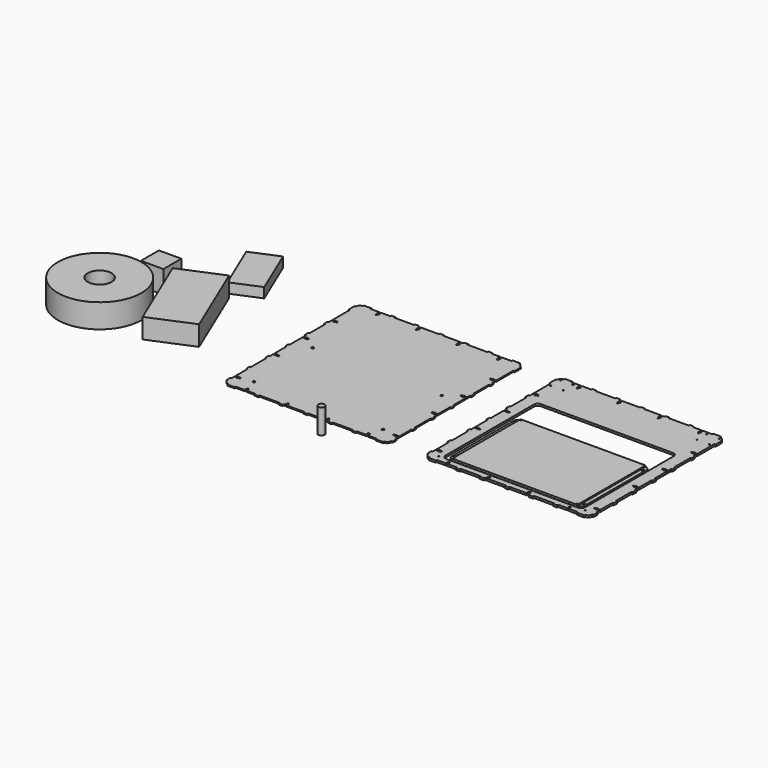
from build123d import *

# Parameters (mm, degrees)
F0_R     = 8
F1_DEPTH = 62
F2_R     = 1.5
F2_R_2   = 50
F2_R_3   = 10
F3_DEPTH = 5
F2_W     = 314
F2_H     = 214
F2_R_4   = 3
F4_DEPTH = 2
F5_DEPTH = 3
F6_DEPTH = 50
F2_R_5   = 105
F2_R_6   = 30
F7_DEPTH = 60
F8_DEPTH = 25
F2_W_2   = 56.4
F2_H_2   = 56.4
F9_DEPTH = 57


with BuildPart() as f1:
    # F0 (on Top) → F1 (new body)
    with BuildSketch(Plane.XY):
        with Locations((-429.197281599, -257.8284740448)):
            Circle(F0_R)
    extrude(amount=F1_DEPTH)


with BuildPart() as f3:
    # F2 (on Top) → F3 (new body)
    with BuildSketch(Plane.XY):
        with BuildLine():
            Line((5, -211.25), (49.3, -211.25))
            Line((49.3, -211.25), (49.3, -208.35))
            Line((49.3, -208.35), (47.8, -208.35))
            Line((47.8, -208.35), (47.8, -205.75))
            Line((47.8, -205.75), (49.3, -205.75))
            Line((49.3, -205.75), (49.3, -202.75))
            Line((49.3, -202.75), (52.7, -202.75))
            Line((52.7, -202.75), (52.7, -205.75))
            Line((52.7, -205.75), (54.2, -205.75))
            Line((54.2, -205.75), (54.2, -208.35))
            Line((54.2, -208.35), (52.7, -208.35))
            Line((52.7, -208.35), (52.7, -211.25))
            Line((52.7, -211.25), (57, -211.25))
            Line((57, -211.25), (57, -214.25))
            Line((57, -214.25), (67, -214.25))
            Line((67, -214.25), (67, -211.25))
            Line((67, -211.25), (117, -211.25))
            Line((117, -211.25), (117, -214.25))
            Line((117, -214.25), (127, -214.25))
            Line((127, -214.25), (127, -211.25))
            Line((127, -211.25), (150.3, -211.25))
            Line((150.3, -211.25), (150.3, -208.35))
            Line((150.3, -208.35), (148.8, -208.35))
            Line((148.8, -208.35), (148.8, -205.75))
            Line((148.8, -205.75), (150.3, -205.75))
            Line((150.3, -205.75), (150.3, -202.75))
            Line((150.3, -202.75), (153.7, -202.75))
            Line((153.7, -202.75), (153.7, -205.75))
            Line((153.7, -205.75), (155.2, -205.75))
            Line((155.2, -205.75), (155.2, -208.35))
            Line((155.2, -208.35), (153.7, -208.35))
            Line((153.7, -208.35), (153.7, -211.25))
            Line((153.7, -211.25), (177, -211.25))
            Line((177, -211.25), (177, -214.25))
            Line((177, -214.25), (195.5, -214.25))
            Line((195.5, -214.25), (195.5, -211.25))
            ThreePointArc((195.5, -211.25), (202.5710678119, -208.3210678119), (205.5, -201.25))
            Line((205.5, -201.25), (208.5, -201.25))
            Line((208.5, -201.25), (208.5, -188.250032))
            Line((208.5, -188.250032), (205.5, -188.250049))
            Line((205.5, -188.250049), (205.5, -179.449994))
            Line((205.5, -179.449994), (199.1, -179.449994))
            Line((199.1, -179.449994), (199.1, -180.949994))
            Line((199.1, -180.949994), (196.5, -180.949994))
            Line((196.5, -180.949994), (196.5, -179.449994))
            Line((196.5, -179.449994), (191.5, -179.449994))
            Line((191.5, -179.449994), (191.5, -176.049994))
            Line((191.5, -176.049994), (196.5, -176.049994))
            Line((196.5, -176.049994), (196.5, -174.549994))
            Line((196.5, -174.549994), (199.1, -174.549994))
            Line((199.1, -174.549994), (199.1, -176.049994))
            Line((199.1, -176.049994), (205.5, -176.049994))
            Line((205.5, -176.049994), (205.5, -138.250065))
            Line((205.5, -138.250065), (208.5, -138.250065))
            Line((208.5, -138.250065), (208.5, -128.250065))
            Line((208.5, -128.250065), (205.5, -128.250065))
            Line((205.5, -128.250065), (205.5, -78.250065))
            Line((205.5, -78.250065), (208.5, -78.250065))
            Line((208.5, -78.250065), (208.5, -68.250065))
            Line((208.5, -68.250065), (205.5, -68.250065))
            Line((205.5, -68.250065), (205.5, -58.449994))
            Line((205.5, -58.449994), (199.1, -58.449994))
            Line((199.1, -58.449994), (199.1, -59.949994))
            Line((199.1, -59.949994), (196.5, -59.949994))
            Line((196.5, -59.949994), (196.5, -58.449994))
            Line((196.5, -58.449994), (191.5, -58.449994))
            Line((191.5, -58.449994), (191.5, -55.049994))
            Line((191.5, -55.049994), (196.5, -55.049994))
            Line((196.5, -55.049994), (196.5, -53.549994))
            Line((196.5, -53.549994), (199.1, -53.549994))
            Line((199.1, -53.549994), (199.1, -55.049994))
            Line((199.1, -55.049994), (205.5, -55.049994))
            Line((205.5, -55.049994), (205.5, -16.250065))
            Line((205.5, -16.250065), (208.5, -16.250065))
            Line((208.5, -16.250065), (208.5, -6.250065))
            Line((208.5, -6.250065), (205.5, -6.250065))
            Line((205.5, -6.250065), (205.5, 33.550006))
            Line((205.5, 33.550006), (199.1, 33.550006))
            Line((199.1, 33.550006), (199.1, 32.050006))
            Line((199.1, 32.050006), (196.5, 32.050006))
            Line((196.5, 32.050006), (196.5, 33.550006))
            Line((196.5, 33.550006), (191.5, 33.550006))
            Line((191.5, 33.550006), (191.5, 36.950006))
            Line((191.5, 36.950006), (196.5, 36.950006))
            Line((196.5, 36.950006), (196.5, 38.450006))
            Line((196.5, 38.450006), (199.1, 38.450006))
            Line((199.1, 38.450006), (199.1, 36.950006))
            Line((199.1, 36.950006), (205.5, 36.950006))
            Line((205.5, 36.950006), (205.5, 45.749935))
            Line((205.5, 45.749935), (208.5, 45.749935))
            Line((208.5, 45.749935), (208.5, 55.749935))
            Line((208.5, 55.749935), (205.5, 55.749935))
            Line((205.5, 55.749935), (205.5, 105.749935))
            Line((205.5, 105.749935), (208.5, 105.749935))
            Line((208.5, 105.749935), (208.5, 115.749935))
            Line((208.5, 115.749935), (205.5, 115.749935))
            Line((205.5, 115.749935), (205.5, 124.550006))
            Line((205.5, 124.550006), (199.1, 124.550006))
            Line((199.1, 124.550006), (199.1, 123.050006))
            Line((199.1, 123.050006), (196.5, 123.050006))
            Line((196.5, 123.050006), (196.5, 124.550006))
            Line((196.5, 124.550006), (191.5, 124.550006))
            Line((191.5, 124.550006), (191.5, 127.950006))
            Line((191.5, 127.950006), (196.5, 127.950006))
            Line((196.5, 127.950006), (196.5, 129.450006))
            Line((196.5, 129.450006), (199.1, 129.450006))
            Line((199.1, 129.450006), (199.1, 127.950006))
            Line((199.1, 127.950006), (205.5, 127.950006))
            Line((205.5, 127.950006), (205.5, 181.25))
            Line((205.5, 181.25), (208.5, 181.25))
            Line((208.5, 181.25), (208.5, 201.25))
            Line((208.5, 201.25), (205.5, 201.25))
            ThreePointArc((205.5, 201.25), (202.5710678119, 208.3210678119), (195.5, 211.25))
            Line((195.5, 211.25), (195.5, 214.25))
            Line((195.5, 214.25), (177, 214.25))
            Line((177, 214.25), (177, 211.25))
            Line((177, 211.25), (153.700002, 211.25))
            Line((153.700002, 211.25), (153.700002, 204.85))
            Line((153.700002, 204.85), (155.200002, 204.85))
            Line((155.200002, 204.85), (155.200002, 202.25))
            Line((155.200002, 202.25), (153.700002, 202.25))
            Line((153.700002, 202.25), (153.700002, 197.25))
            Line((153.700002, 197.25), (150.300002, 197.25))
            Line((150.300002, 197.25), (150.300002, 202.25))
            Line((150.300002, 202.25), (148.800002, 202.25))
            Line((148.800002, 202.25), (148.800002, 204.85))
            Line((148.800002, 204.85), (150.300002, 204.85))
            Line((150.300002, 204.85), (150.300002, 211.25))
            Line((150.300002, 211.25), (127, 211.25))
            Line((127, 211.25), (127, 214.25))
            Line((127, 214.25), (117, 214.25))
            Line((117, 214.25), (117, 211.25))
            Line((117, 211.25), (67, 211.25))
            Line((67, 211.25), (67, 214.25))
            Line((67, 214.25), (57, 214.25))
            Line((57, 214.25), (57, 211.25))
            Line((57, 211.25), (52.700002, 211.25))
            Line((52.700002, 211.25), (52.700002, 204.85))
            Line((52.700002, 204.85), (54.200002, 204.85))
            Line((54.200002, 204.85), (54.200002, 202.25))
            Line((54.200002, 202.25), (52.700002, 202.25))
            Line((52.700002, 202.25), (52.700002, 197.25))
            Line((52.700002, 197.25), (49.300002, 197.25))
            Line((49.300002, 197.25), (49.300002, 202.25))
            Line((49.300002, 202.25), (47.800002, 202.25))
            Line((47.800002, 202.25), (47.800002, 204.85))
            Line((47.800002, 204.85), (49.300002, 204.85))
            Line((49.300002, 204.85), (49.300002, 211.25))
            Line((49.300002, 211.25), (5, 211.25))
            Line((5, 211.25), (5, 214.25))
            Line((5, 214.25), (-5, 214.25))
            Line((-5, 214.25), (-5, 211.25))
            Line((-5, 211.25), (-49.299998, 211.25))
            Line((-49.299998, 211.25), (-49.299998, 204.85))
            Line((-49.299998, 204.85), (-47.799998, 204.85))
            Line((-47.799998, 204.85), (-47.799998, 202.25))
            Line((-47.799998, 202.25), (-49.299998, 202.25))
            Line((-49.299998, 202.25), (-49.299998, 197.25))
            Line((-49.299998, 197.25), (-52.699998, 197.25))
            Line((-52.699998, 197.25), (-52.699998, 202.25))
            Line((-52.699998, 202.25), (-54.199998, 202.25))
            Line((-54.199998, 202.25), (-54.199998, 204.85))
            Line((-54.199998, 204.85), (-52.699998, 204.85))
            Line((-52.699998, 204.85), (-52.699998, 211.25))
            Line((-52.699998, 211.25), (-57, 211.25))
            Line((-57, 211.25), (-57, 214.25))
            Line((-57, 214.25), (-67, 214.25))
            Line((-67, 214.25), (-67, 211.25))
            Line((-67, 211.25), (-117, 211.25))
            Line((-117, 211.25), (-117, 214.25))
            Line((-117, 214.25), (-127, 214.25))
            Line((-127, 214.25), (-127, 211.25))
            Line((-127, 211.25), (-150.299998, 211.25))
            Line((-150.299998, 211.25), (-150.299998, 204.85))
            Line((-150.299998, 204.85), (-148.799998, 204.85))
            Line((-148.799998, 204.85), (-148.799998, 202.25))
            Line((-148.799998, 202.25), (-150.299998, 202.25))
            Line((-150.299998, 202.25), (-150.299998, 197.25))
            Line((-150.299998, 197.25), (-153.699998, 197.25))
            Line((-153.699998, 197.25), (-153.699998, 202.25))
            Line((-153.699998, 202.25), (-155.199998, 202.25))
            Line((-155.199998, 202.25), (-155.199998, 204.85))
            Line((-155.199998, 204.85), (-153.699998, 204.85))
            Line((-153.699998, 204.85), (-153.699998, 211.25))
            Line((-153.699998, 211.25), (-177, 211.25))
            Line((-177, 211.25), (-177, 214.25))
            Line((-177, 214.25), (-195.5, 214.25))
            Line((-195.5, 214.25), (-195.5, 211.25))
            ThreePointArc((-195.5, 211.25), (-202.5710678119, 208.3210678119), (-205.5, 201.25))
            Line((-205.5, 201.25), (-208.5, 201.25))
            Line((-208.5, 201.25), (-208.5, 181.25))
            Line((-208.5, 181.25), (-205.5, 181.25))
            Line((-205.5, 181.25), (-205.5, 127.950006))
            Line((-205.5, 127.950006), (-199.1, 127.950006))
            Line((-199.1, 127.950006), (-199.1, 129.450006))
            Line((-199.1, 129.450006), (-196.5, 129.450006))
            Line((-196.5, 129.450006), (-196.5, 127.950006))
            Line((-196.5, 127.950006), (-191.5, 127.950006))
            Line((-191.5, 127.950006), (-191.5, 124.550006))
            Line((-191.5, 124.550006), (-196.5, 124.550006))
            Line((-196.5, 124.550006), (-196.5, 123.050006))
            Line((-196.5, 123.050006), (-199.1, 123.050006))
            Line((-199.1, 123.050006), (-199.1, 124.550006))
            Line((-199.1, 124.550006), (-205.5, 124.550006))
            Line((-205.5, 124.550006), (-205.5, 115.749935))
            Line((-205.5, 115.749935), (-208.5, 115.749935))
            Line((-208.5, 115.749935), (-208.5, 105.749935))
            Line((-208.5, 105.749935), (-205.5, 105.749935))
            Line((-205.5, 105.749935), (-205.5, 55.749935))
            Line((-205.5, 55.749935), (-208.5, 55.749935))
            Line((-208.5, 55.749935), (-208.5, 45.749935))
            Line((-208.5, 45.749935), (-205.5, 45.749935))
            Line((-205.5, 45.749935), (-205.5, 36.950006))
            Line((-205.5, 36.950006), (-199.1, 36.950006))
            Line((-199.1, 36.950006), (-199.1, 38.450006))
            Line((-199.1, 38.450006), (-196.5, 38.450006))
            Line((-196.5, 38.450006), (-196.5, 36.950006))
            Line((-196.5, 36.950006), (-191.5, 36.950006))
            Line((-191.5, 36.950006), (-191.5, 33.550006))
            Line((-191.5, 33.550006), (-196.5, 33.550006))
            Line((-196.5, 33.550006), (-196.5, 32.050006))
            Line((-196.5, 32.050006), (-199.1, 32.050006))
            Line((-199.1, 32.050006), (-199.1, 33.550006))
            Line((-199.1, 33.550006), (-205.5, 33.550006))
            Line((-205.5, 33.550006), (-205.5, -6.250065))
            Line((-205.5, -6.250065), (-208.5, -6.250065))
            Line((-208.5, -6.250065), (-208.5, -16.250065))
            Line((-208.5, -16.250065), (-205.5, -16.250065))
            Line((-205.5, -16.250065), (-205.5, -55.049994))
            Line((-205.5, -55.049994), (-199.1, -55.049994))
            Line((-199.1, -55.049994), (-199.1, -53.549994))
            Line((-199.1, -53.549994), (-196.5, -53.549994))
            Line((-196.5, -53.549994), (-196.5, -55.049994))
            Line((-196.5, -55.049994), (-191.5, -55.049994))
            Line((-191.5, -55.049994), (-191.5, -58.449994))
            Line((-191.5, -58.449994), (-196.5, -58.449994))
            Line((-196.5, -58.449994), (-196.5, -59.949994))
            Line((-196.5, -59.949994), (-199.1, -59.949994))
            Line((-199.1, -59.949994), (-199.1, -58.449994))
            Line((-199.1, -58.449994), (-205.5, -58.449994))
            Line((-205.5, -58.449994), (-205.5, -68.250065))
            Line((-205.5, -68.250065), (-208.5, -68.250065))
            Line((-208.5, -68.250065), (-208.5, -78.250065))
            Line((-208.5, -78.250065), (-205.5, -78.250065))
            Line((-205.5, -78.250065), (-205.5, -128.250065))
            Line((-205.5, -128.250065), (-208.5, -128.250065))
            Line((-208.5, -128.250065), (-208.5, -138.250065))
            Line((-208.5, -138.250065), (-205.5, -138.250065))
            Line((-205.5, -138.250065), (-205.5, -176.049994))
            Line((-205.5, -176.049994), (-199.1, -176.049994))
            Line((-199.1, -176.049994), (-199.1, -174.549994))
            Line((-199.1, -174.549994), (-196.5, -174.549994))
            Line((-196.5, -174.549994), (-196.5, -176.049994))
            Line((-196.5, -176.049994), (-191.5, -176.049994))
            Line((-191.5, -176.049994), (-191.5, -179.449994))
            Line((-191.5, -179.449994), (-196.5, -179.449994))
            Line((-196.5, -179.449994), (-196.5, -180.949994))
            Line((-196.5, -180.949994), (-199.1, -180.949994))
            Line((-199.1, -180.949994), (-199.1, -179.449994))
            Line((-199.1, -179.449994), (-205.5, -179.449994))
            Line((-205.5, -179.449994), (-205.5, -188.250049))
            Line((-205.5, -188.250049), (-208.5, -188.250032))
            Line((-208.5, -188.250032), (-208.5, -201.25))
            Line((-208.5, -201.25), (-205.5, -201.25))
            ThreePointArc((-205.5, -201.25), (-202.5710678119, -208.3210678119), (-195.5, -211.25))
            Line((-195.5, -211.25), (-195.5, -214.25))
            Line((-195.5, -214.25), (-177, -214.25))
            Line((-177, -214.25), (-177, -211.25))
            Line((-177, -211.25), (-153.7, -211.25))
            Line((-153.7, -211.25), (-153.7, -208.35))
            Line((-153.7, -208.35), (-155.2, -208.35))
            Line((-155.2, -208.35), (-155.2, -205.75))
            Line((-155.2, -205.75), (-153.7, -205.75))
            Line((-153.7, -205.75), (-153.7, -202.75))
            Line((-153.7, -202.75), (-150.3, -202.75))
            Line((-150.3, -202.75), (-150.3, -205.75))
            Line((-150.3, -205.75), (-148.8, -205.75))
            Line((-148.8, -205.75), (-148.8, -208.35))
            Line((-148.8, -208.35), (-150.3, -208.35))
            Line((-150.3, -208.35), (-150.3, -211.25))
            Line((-150.3, -211.25), (-127, -211.25))
            Line((-127, -211.25), (-127, -214.25))
            Line((-127, -214.25), (-117, -214.25))
            Line((-117, -214.25), (-117, -211.25))
            Line((-117, -211.25), (-67, -211.25))
            Line((-67, -211.25), (-67, -214.25))
            Line((-67, -214.25), (-57, -214.25))
            Line((-57, -214.25), (-57, -211.25))
            Line((-57, -211.25), (-52.7, -211.25))
            Line((-52.7, -211.25), (-52.7, -208.35))
            Line((-52.7, -208.35), (-54.2, -208.35))
            Line((-54.2, -208.35), (-54.2, -205.75))
            Line((-54.2, -205.75), (-52.7, -205.75))
            Line((-52.7, -205.75), (-52.7, -202.75))
            Line((-52.7, -202.75), (-49.3, -202.75))
            Line((-49.3, -202.75), (-49.3, -205.75))
            Line((-49.3, -205.75), (-47.8, -205.75))
            Line((-47.8, -205.75), (-47.8, -208.35))
            Line((-47.8, -208.35), (-49.3, -208.35))
            Line((-49.3, -208.35), (-49.3, -211.25))
            Line((-49.3, -211.25), (-5, -211.25))
            Line((-5, -211.25), (-5, -214.25))
            Line((-5, -214.25), (5, -214.25))
            Line((5, -214.25), (5, -211.25))
        make_face()
        with Locations((-183.5, -196.25)):
            Circle(F2_R, mode=Mode.SUBTRACT)
        with Locations((183.5, -196.25)):
            Circle(F2_R, mode=Mode.SUBTRACT)
        with BuildLine():
            ThreePointArc((175.5, -186.25), (172.5710678119, -193.3210678119), (165.5, -196.25))
            Line((165.5, -196.25), (-165.5, -196.25))
            ThreePointArc((-165.5, -196.25), (-172.5710678119, -193.3210678119), (-175.5, -186.25))
            Line((-175.5, -186.25), (-175.5, 91.25))
            ThreePointArc((-175.5, 91.25), (-172.5710678119, 98.3210678119), (-165.5, 101.25))
            Line((-165.5, 101.25), (165.5, 101.25))
            ThreePointArc((165.5, 101.25), (172.5710678119, 98.3210678119), (175.5, 91.25))
            Line((175.5, 91.25), (175.5, -186.25))
        make_face(mode=Mode.SUBTRACT)
        with Locations((-199, 173.75)):
            Circle(F2_R, mode=Mode.SUBTRACT)
        with Locations((-168, 173.75)):
            Circle(F2_R, mode=Mode.SUBTRACT)
        with Locations((-199, 204.75)):
            Circle(F2_R, mode=Mode.SUBTRACT)
        with Locations((-168, 204.75)):
            Circle(F2_R, mode=Mode.SUBTRACT)
        with Locations((-107.5, 156.25)):
            Circle(F2_R_2, mode=Mode.SUBTRACT)
        with Locations((0, 156.25)):
            Circle(F2_R_2, mode=Mode.SUBTRACT)
        with Locations((107.5, 156.25)):
            Circle(F2_R_2, mode=Mode.SUBTRACT)
        with Locations((168, 173.75)):
            Circle(F2_R, mode=Mode.SUBTRACT)
        with Locations((199, 173.75)):
            Circle(F2_R, mode=Mode.SUBTRACT)
        with Locations((168, 204.75)):
            Circle(F2_R, mode=Mode.SUBTRACT)
        with Locations((199, 204.75)):
            Circle(F2_R, mode=Mode.SUBTRACT)
        with Locations((-107.5, 156.25)):
            Circle(F2_R_2)
        with Locations((-107.5, 156.25)):
            Circle(F2_R_3, mode=Mode.SUBTRACT)
        with Locations((107.5, 156.25)):
            Circle(F2_R_2)
        with Locations((107.5, 156.25)):
            Circle(F2_R_3, mode=Mode.SUBTRACT)
        with Locations((0, 156.25)):
            Circle(F2_R_2)
        with Locations((0, 156.25)):
            Circle(F2_R_3, mode=Mode.SUBTRACT)
        with Locations((-107.5, 156.25)):
            Circle(F2_R_3)
        with Locations((0, 156.25)):
            Circle(F2_R_3)
        with Locations((107.5, 156.25)):
            Circle(F2_R_3)
    extrude(amount=F3_DEPTH)


with BuildPart() as f3b:
    # F2 (on Top) → F3, piece 2 (new body)
    with BuildSketch(Plane.XY):
        with Locations((0, -80.75)):
            Rectangle(F2_W, F2_H)
        with Locations((-154.5, -185.25)):
            Circle(F2_R, mode=Mode.SUBTRACT)
        with Locations((154.5, -185.25)):
            Circle(F2_R, mode=Mode.SUBTRACT)
        with Locations((-154.5, 23.75)):
            Circle(F2_R, mode=Mode.SUBTRACT)
        with Locations((154.5, 23.75)):
            Circle(F2_R, mode=Mode.SUBTRACT)
    extrude(amount=F3_DEPTH)

    # F2 (on Top) → F4 (join)
    with BuildSketch(Plane.XY):
        with BuildLine():
            ThreePointArc((-157, 26.25), (-164.0710678119, 23.3210678119), (-167, 16.25))
            Line((-167, 16.25), (-167, -177.75))
            ThreePointArc((-167, -177.75), (-164.0710678119, -184.8210678119), (-157, -187.75))
            Line((-157, -187.75), (-157, 26.25))
        make_face()
        with Locations((-162, -172.75)):
            Circle(F2_R_4, mode=Mode.SUBTRACT)
        with Locations((-162, 11.25)):
            Circle(F2_R_4, mode=Mode.SUBTRACT)
        with BuildLine():
            ThreePointArc((167, 16.25), (164.0710678119, 23.3210678119), (157, 26.25))
            Line((157, 26.25), (157, -187.75))
            ThreePointArc((157, -187.75), (164.0710678119, -184.8210678119), (167, -177.75))
            Line((167, -177.75), (167, 16.25))
        make_face()
        with Locations((162, -172.75)):
            Circle(F2_R_4, mode=Mode.SUBTRACT)
        with Locations((162, 11.25)):
            Circle(F2_R_4, mode=Mode.SUBTRACT)
    extrude(amount=F4_DEPTH)


with BuildPart() as f5:
    # F2 (on Top) → F5 (new body)
    with BuildSketch(Plane.XY):
        with BuildLine():
            Line((-499.6031921292, -211.2499983311), (-455.3031921292, -211.2499983311))
            Line((-455.3031921292, -211.2499983311), (-455.3031921292, -208.3499983311))
            Line((-455.3031921292, -208.3499983311), (-456.8031921292, -208.3499983311))
            Line((-456.8031921292, -208.3499983311), (-456.8031921292, -205.7499983311))
            Line((-456.8031921292, -205.7499983311), (-455.3031921292, -205.7499983311))
            Line((-455.3031921292, -205.7499983311), (-455.3031921292, -202.7499983311))
            Line((-455.3031921292, -202.7499983311), (-451.9031921292, -202.7499983311))
            Line((-451.9031921292, -202.7499983311), (-451.9031921292, -205.7499983311))
            Line((-451.9031921292, -205.7499983311), (-450.4031921292, -205.7499983311))
            Line((-450.4031921292, -205.7499983311), (-450.4031921292, -208.3499983311))
            Line((-450.4031921292, -208.3499983311), (-451.9031921292, -208.3499983311))
            Line((-451.9031921292, -208.3499983311), (-451.9031921292, -211.2499983311))
            Line((-451.9031921292, -211.2499983311), (-447.6031921292, -211.2499983311))
            Line((-447.6031921292, -211.2499983311), (-447.6031921292, -214.2499983311))
            Line((-447.6031921292, -214.2499983311), (-437.6031921292, -214.2499983311))
            Line((-437.6031921292, -214.2499983311), (-437.6031921292, -211.2499983311))
            Line((-437.6031921292, -211.2499983311), (-387.6031921292, -211.2499983311))
            Line((-387.6031921292, -211.2499983311), (-387.6031921292, -214.2499983311))
            Line((-387.6031921292, -214.2499983311), (-377.6031921292, -214.2499983311))
            Line((-377.6031921292, -214.2499983311), (-377.6031921292, -211.2499983311))
            Line((-377.6031921292, -211.2499983311), (-354.3031921292, -211.2499983311))
            Line((-354.3031921292, -211.2499983311), (-354.3031921292, -208.3499983311))
            Line((-354.3031921292, -208.3499983311), (-355.8031921292, -208.3499983311))
            Line((-355.8031921292, -208.3499983311), (-355.8031921292, -205.7499983311))
            Line((-355.8031921292, -205.7499983311), (-354.3031921292, -205.7499983311))
            Line((-354.3031921292, -205.7499983311), (-354.3031921292, -202.7499983311))
            Line((-354.3031921292, -202.7499983311), (-350.9031921292, -202.7499983311))
            Line((-350.9031921292, -202.7499983311), (-350.9031921292, -205.7499983311))
            Line((-350.9031921292, -205.7499983311), (-349.4031921292, -205.7499983311))
            Line((-349.4031921292, -205.7499983311), (-349.4031921292, -208.3499983311))
            Line((-349.4031921292, -208.3499983311), (-350.9031921292, -208.3499983311))
            Line((-350.9031921292, -208.3499983311), (-350.9031921292, -211.2499983311))
            Line((-350.9031921292, -211.2499983311), (-327.6031921292, -211.2499983311))
            Line((-327.6031921292, -211.2499983311), (-327.6031921292, -214.2499983311))
            Line((-327.6031921292, -214.2499983311), (-309.1031921292, -214.2499983311))
            Line((-309.1031921292, -214.2499983311), (-309.1031921292, -211.2499983311))
            ThreePointArc((-309.1031921292, -211.2499983311), (-302.0321243174, -208.3210661429), (-299.1031921292, -201.2499983311))
            Line((-299.1031921292, -201.2499983311), (-296.1031921292, -201.2499983311))
            Line((-296.1031921292, -201.2499983311), (-296.1031921292, -188.2500303311))
            Line((-296.1031921292, -188.2500303311), (-299.1031921292, -188.2500473311))
            Line((-299.1031921292, -188.2500473311), (-299.1031921292, -179.4499923311))
            Line((-299.1031921292, -179.4499923311), (-305.5031921292, -179.4499923311))
            Line((-305.5031921292, -179.4499923311), (-305.5031921292, -180.9499923311))
            Line((-305.5031921292, -180.9499923311), (-308.1031921292, -180.9499923311))
            Line((-308.1031921292, -180.9499923311), (-308.1031921292, -179.4499923311))
            Line((-308.1031921292, -179.4499923311), (-313.1031921292, -179.4499923311))
            Line((-313.1031921292, -179.4499923311), (-313.1031921292, -176.0499923311))
            Line((-313.1031921292, -176.0499923311), (-308.1031921292, -176.0499923311))
            Line((-308.1031921292, -176.0499923311), (-308.1031921292, -174.5499923311))
            Line((-308.1031921292, -174.5499923311), (-305.5031921292, -174.5499923311))
            Line((-305.5031921292, -174.5499923311), (-305.5031921292, -176.0499923311))
            Line((-305.5031921292, -176.0499923311), (-299.1031921292, -176.0499923311))
            Line((-299.1031921292, -176.0499923311), (-299.1031921292, -138.2500633311))
            Line((-299.1031921292, -138.2500633311), (-296.1031921292, -138.2500633311))
            Line((-296.1031921292, -138.2500633311), (-296.1031921292, -128.2500633311))
            Line((-296.1031921292, -128.2500633311), (-299.1031921292, -128.2500633311))
            Line((-299.1031921292, -128.2500633311), (-299.1031921292, -78.2500633311))
            Line((-299.1031921292, -78.2500633311), (-296.1031921292, -78.2500633311))
            Line((-296.1031921292, -78.2500633311), (-296.1031921292, -68.2500633311))
            Line((-296.1031921292, -68.2500633311), (-299.1031921292, -68.2500633311))
            Line((-299.1031921292, -68.2500633311), (-299.1031921292, -58.4499923311))
            Line((-299.1031921292, -58.4499923311), (-305.5031921292, -58.4499923311))
            Line((-305.5031921292, -58.4499923311), (-305.5031921292, -59.9499923311))
            Line((-305.5031921292, -59.9499923311), (-308.1031921292, -59.9499923311))
            Line((-308.1031921292, -59.9499923311), (-308.1031921292, -58.4499923311))
            Line((-308.1031921292, -58.4499923311), (-313.1031921292, -58.4499923311))
            Line((-313.1031921292, -58.4499923311), (-313.1031921292, -55.0499923311))
            Line((-313.1031921292, -55.0499923311), (-308.1031921292, -55.0499923311))
            Line((-308.1031921292, -55.0499923311), (-308.1031921292, -53.5499923311))
            Line((-308.1031921292, -53.5499923311), (-305.5031921292, -53.5499923311))
            Line((-305.5031921292, -53.5499923311), (-305.5031921292, -55.0499923311))
            Line((-305.5031921292, -55.0499923311), (-299.1031921292, -55.0499923311))
            Line((-299.1031921292, -55.0499923311), (-299.1031921292, -16.2500633311))
            Line((-299.1031921292, -16.2500633311), (-296.1031921292, -16.2500633311))
            Line((-296.1031921292, -16.2500633311), (-296.1031921292, -6.2500633311))
            Line((-296.1031921292, -6.2500633311), (-299.1031921292, -6.2500633311))
            Line((-299.1031921292, -6.2500633311), (-299.1031921292, 33.5500076689))
            Line((-299.1031921292, 33.5500076689), (-305.5031921292, 33.5500076689))
            Line((-305.5031921292, 33.5500076689), (-305.5031921292, 32.0500076689))
            Line((-305.5031921292, 32.0500076689), (-308.1031921292, 32.0500076689))
            Line((-308.1031921292, 32.0500076689), (-308.1031921292, 33.5500076689))
            Line((-308.1031921292, 33.5500076689), (-313.1031921292, 33.5500076689))
            Line((-313.1031921292, 33.5500076689), (-313.1031921292, 36.9500076689))
            Line((-313.1031921292, 36.9500076689), (-308.1031921292, 36.9500076689))
            Line((-308.1031921292, 36.9500076689), (-308.1031921292, 38.4500076689))
            Line((-308.1031921292, 38.4500076689), (-305.5031921292, 38.4500076689))
            Line((-305.5031921292, 38.4500076689), (-305.5031921292, 36.9500076689))
            Line((-305.5031921292, 36.9500076689), (-299.1031921292, 36.9500076689))
            Line((-299.1031921292, 36.9500076689), (-299.1031921292, 45.7499366689))
            Line((-299.1031921292, 45.7499366689), (-296.1031921292, 45.7499366689))
            Line((-296.1031921292, 45.7499366689), (-296.1031921292, 55.7499366689))
            Line((-296.1031921292, 55.7499366689), (-299.1031921292, 55.7499366689))
            Line((-299.1031921292, 55.7499366689), (-299.1031921292, 105.7499366689))
            Line((-299.1031921292, 105.7499366689), (-296.1031921292, 105.7499366689))
            Line((-296.1031921292, 105.7499366689), (-296.1031921292, 115.7499366689))
            Line((-296.1031921292, 115.7499366689), (-299.1031921292, 115.7499366689))
            Line((-299.1031921292, 115.7499366689), (-299.1031921292, 124.5500076689))
            Line((-299.1031921292, 124.5500076689), (-305.5031921292, 124.5500076689))
            Line((-305.5031921292, 124.5500076689), (-305.5031921292, 123.0500076689))
            Line((-305.5031921292, 123.0500076689), (-308.1031921292, 123.0500076689))
            Line((-308.1031921292, 123.0500076689), (-308.1031921292, 124.5500076689))
            Line((-308.1031921292, 124.5500076689), (-313.1031921292, 124.5500076689))
            Line((-313.1031921292, 124.5500076689), (-313.1031921292, 127.9500076689))
            Line((-313.1031921292, 127.9500076689), (-308.1031921292, 127.9500076689))
            Line((-308.1031921292, 127.9500076689), (-308.1031921292, 129.4500076689))
            Line((-308.1031921292, 129.4500076689), (-305.5031921292, 129.4500076689))
            Line((-305.5031921292, 129.4500076689), (-305.5031921292, 127.9500076689))
            Line((-305.5031921292, 127.9500076689), (-299.1031921292, 127.9500076689))
            Line((-299.1031921292, 127.9500076689), (-299.1031921292, 181.2500016689))
            Line((-299.1031921292, 181.2500016689), (-296.1031921292, 181.2500016689))
            Line((-296.1031921292, 181.2500016689), (-296.1031921292, 201.2500016689))
            Line((-296.1031921292, 201.2500016689), (-299.1031921292, 201.2500016689))
            ThreePointArc((-299.1031921292, 201.2500016689), (-302.0321243174, 208.3210694808), (-309.1031921292, 211.2500016689))
            Line((-309.1031921292, 211.2500016689), (-309.1031921292, 214.2500016689))
            Line((-309.1031921292, 214.2500016689), (-327.6031921292, 214.2500016689))
            Line((-327.6031921292, 214.2500016689), (-327.6031921292, 211.2500016689))
            Line((-327.6031921292, 211.2500016689), (-350.9031901292, 211.2500016689))
            Line((-350.9031901292, 211.2500016689), (-350.9031901292, 204.8500016689))
            Line((-350.9031901292, 204.8500016689), (-349.4031901292, 204.8500016689))
            Line((-349.4031901292, 204.8500016689), (-349.4031901292, 202.2500016689))
            Line((-349.4031901292, 202.2500016689), (-350.9031901292, 202.2500016689))
            Line((-350.9031901292, 202.2500016689), (-350.9031901292, 197.2500016689))
            Line((-350.9031901292, 197.2500016689), (-354.3031901292, 197.2500016689))
            Line((-354.3031901292, 197.2500016689), (-354.3031901292, 202.2500016689))
            Line((-354.3031901292, 202.2500016689), (-355.8031901292, 202.2500016689))
            Line((-355.8031901292, 202.2500016689), (-355.8031901292, 204.8500016689))
            Line((-355.8031901292, 204.8500016689), (-354.3031901292, 204.8500016689))
            Line((-354.3031901292, 204.8500016689), (-354.3031901292, 211.2500016689))
            Line((-354.3031901292, 211.2500016689), (-377.6031921292, 211.2500016689))
            Line((-377.6031921292, 211.2500016689), (-377.6031921292, 214.2500016689))
            Line((-377.6031921292, 214.2500016689), (-387.6031921292, 214.2500016689))
            Line((-387.6031921292, 214.2500016689), (-387.6031921292, 211.2500016689))
            Line((-387.6031921292, 211.2500016689), (-437.6031921292, 211.2500016689))
            Line((-437.6031921292, 211.2500016689), (-437.6031921292, 214.2500016689))
            Line((-437.6031921292, 214.2500016689), (-447.6031921292, 214.2500016689))
            Line((-447.6031921292, 214.2500016689), (-447.6031921292, 211.2500016689))
            Line((-447.6031921292, 211.2500016689), (-451.9031901292, 211.2500016689))
            Line((-451.9031901292, 211.2500016689), (-451.9031901292, 204.8500016689))
            Line((-451.9031901292, 204.8500016689), (-450.4031901292, 204.8500016689))
            Line((-450.4031901292, 204.8500016689), (-450.4031901292, 202.2500016689))
            Line((-450.4031901292, 202.2500016689), (-451.9031901292, 202.2500016689))
            Line((-451.9031901292, 202.2500016689), (-451.9031901292, 197.2500016689))
            Line((-451.9031901292, 197.2500016689), (-455.3031901292, 197.2500016689))
            Line((-455.3031901292, 197.2500016689), (-455.3031901292, 202.2500016689))
            Line((-455.3031901292, 202.2500016689), (-456.8031901292, 202.2500016689))
            Line((-456.8031901292, 202.2500016689), (-456.8031901292, 204.8500016689))
            Line((-456.8031901292, 204.8500016689), (-455.3031901292, 204.8500016689))
            Line((-455.3031901292, 204.8500016689), (-455.3031901292, 211.2500016689))
            Line((-455.3031901292, 211.2500016689), (-499.6031921292, 211.2500016689))
            Line((-499.6031921292, 211.2500016689), (-499.6031921292, 214.2500016689))
            Line((-499.6031921292, 214.2500016689), (-509.6031921292, 214.2500016689))
            Line((-509.6031921292, 214.2500016689), (-509.6031921292, 211.2500016689))
            Line((-509.6031921292, 211.2500016689), (-553.9031901292, 211.2500016689))
            Line((-553.9031901292, 211.2500016689), (-553.9031901292, 204.8500016689))
            Line((-553.9031901292, 204.8500016689), (-552.4031901292, 204.8500016689))
            Line((-552.4031901292, 204.8500016689), (-552.4031901292, 202.2500016689))
            Line((-552.4031901292, 202.2500016689), (-553.9031901292, 202.2500016689))
            Line((-553.9031901292, 202.2500016689), (-553.9031901292, 197.2500016689))
            Line((-553.9031901292, 197.2500016689), (-557.3031901292, 197.2500016689))
            Line((-557.3031901292, 197.2500016689), (-557.3031901292, 202.2500016689))
            Line((-557.3031901292, 202.2500016689), (-558.8031901292, 202.2500016689))
            Line((-558.8031901292, 202.2500016689), (-558.8031901292, 204.8500016689))
            Line((-558.8031901292, 204.8500016689), (-557.3031901292, 204.8500016689))
            Line((-557.3031901292, 204.8500016689), (-557.3031901292, 211.2500016689))
            Line((-557.3031901292, 211.2500016689), (-561.6031921292, 211.2500016689))
            Line((-561.6031921292, 211.2500016689), (-561.6031921292, 214.2500016689))
            Line((-561.6031921292, 214.2500016689), (-571.6031921292, 214.2500016689))
            Line((-571.6031921292, 214.2500016689), (-571.6031921292, 211.2500016689))
            Line((-571.6031921292, 211.2500016689), (-621.6031921292, 211.2500016689))
            Line((-621.6031921292, 211.2500016689), (-621.6031921292, 214.2500016689))
            Line((-621.6031921292, 214.2500016689), (-631.6031921292, 214.2500016689))
            Line((-631.6031921292, 214.2500016689), (-631.6031921292, 211.2500016689))
            Line((-631.6031921292, 211.2500016689), (-654.9031901292, 211.2500016689))
            Line((-654.9031901292, 211.2500016689), (-654.9031901292, 204.8500016689))
            Line((-654.9031901292, 204.8500016689), (-653.4031901292, 204.8500016689))
            Line((-653.4031901292, 204.8500016689), (-653.4031901292, 202.2500016689))
            Line((-653.4031901292, 202.2500016689), (-654.9031901292, 202.2500016689))
            Line((-654.9031901292, 202.2500016689), (-654.9031901292, 197.2500016689))
            Line((-654.9031901292, 197.2500016689), (-658.3031901292, 197.2500016689))
            Line((-658.3031901292, 197.2500016689), (-658.3031901292, 202.2500016689))
            Line((-658.3031901292, 202.2500016689), (-659.8031901292, 202.2500016689))
            Line((-659.8031901292, 202.2500016689), (-659.8031901292, 204.8500016689))
            Line((-659.8031901292, 204.8500016689), (-658.3031901292, 204.8500016689))
            Line((-658.3031901292, 204.8500016689), (-658.3031901292, 211.2500016689))
            Line((-658.3031901292, 211.2500016689), (-681.6031921292, 211.2500016689))
            Line((-681.6031921292, 211.2500016689), (-681.6031921292, 214.2500016689))
            Line((-681.6031921292, 214.2500016689), (-700.1031921292, 214.2500016689))
            Line((-700.1031921292, 214.2500016689), (-700.1031921292, 211.2500016689))
            ThreePointArc((-700.1031921292, 211.2500016689), (-707.1742599411, 208.3210694808), (-710.1031921292, 201.2500016689))
            Line((-710.1031921292, 201.2500016689), (-713.1031921292, 201.2500016689))
            Line((-713.1031921292, 201.2500016689), (-713.1031921292, 181.2500016689))
            Line((-713.1031921292, 181.2500016689), (-710.1031921292, 181.2500016689))
            Line((-710.1031921292, 181.2500016689), (-710.1031921292, 127.9500076689))
            Line((-710.1031921292, 127.9500076689), (-703.7031921292, 127.9500076689))
            Line((-703.7031921292, 127.9500076689), (-703.7031921292, 129.4500076689))
            Line((-703.7031921292, 129.4500076689), (-701.1031921292, 129.4500076689))
            Line((-701.1031921292, 129.4500076689), (-701.1031921292, 127.9500076689))
            Line((-701.1031921292, 127.9500076689), (-696.1031921292, 127.9500076689))
            Line((-696.1031921292, 127.9500076689), (-696.1031921292, 124.5500076689))
            Line((-696.1031921292, 124.5500076689), (-701.1031921292, 124.5500076689))
            Line((-701.1031921292, 124.5500076689), (-701.1031921292, 123.0500076689))
            Line((-701.1031921292, 123.0500076689), (-703.7031921292, 123.0500076689))
            Line((-703.7031921292, 123.0500076689), (-703.7031921292, 124.5500076689))
            Line((-703.7031921292, 124.5500076689), (-710.1031921292, 124.5500076689))
            Line((-710.1031921292, 124.5500076689), (-710.1031921292, 115.7499366689))
            Line((-710.1031921292, 115.7499366689), (-713.1031921292, 115.7499366689))
            Line((-713.1031921292, 115.7499366689), (-713.1031921292, 105.7499366689))
            Line((-713.1031921292, 105.7499366689), (-710.1031921292, 105.7499366689))
            Line((-710.1031921292, 105.7499366689), (-710.1031921292, 55.7499366689))
            Line((-710.1031921292, 55.7499366689), (-713.1031921292, 55.7499366689))
            Line((-713.1031921292, 55.7499366689), (-713.1031921292, 45.7499366689))
            Line((-713.1031921292, 45.7499366689), (-710.1031921292, 45.7499366689))
            Line((-710.1031921292, 45.7499366689), (-710.1031921292, 36.9500076689))
            Line((-710.1031921292, 36.9500076689), (-703.7031921292, 36.9500076689))
            Line((-703.7031921292, 36.9500076689), (-703.7031921292, 38.4500076689))
            Line((-703.7031921292, 38.4500076689), (-701.1031921292, 38.4500076689))
            Line((-701.1031921292, 38.4500076689), (-701.1031921292, 36.9500076689))
            Line((-701.1031921292, 36.9500076689), (-696.1031921292, 36.9500076689))
            Line((-696.1031921292, 36.9500076689), (-696.1031921292, 33.5500076689))
            Line((-696.1031921292, 33.5500076689), (-701.1031921292, 33.5500076689))
            Line((-701.1031921292, 33.5500076689), (-701.1031921292, 32.0500076689))
            Line((-701.1031921292, 32.0500076689), (-703.7031921292, 32.0500076689))
            Line((-703.7031921292, 32.0500076689), (-703.7031921292, 33.5500076689))
            Line((-703.7031921292, 33.5500076689), (-710.1031921292, 33.5500076689))
            Line((-710.1031921292, 33.5500076689), (-710.1031921292, -6.2500633311))
            Line((-710.1031921292, -6.2500633311), (-713.1031921292, -6.2500633311))
            Line((-713.1031921292, -6.2500633311), (-713.1031921292, -16.2500633311))
            Line((-713.1031921292, -16.2500633311), (-710.1031921292, -16.2500633311))
            Line((-710.1031921292, -16.2500633311), (-710.1031921292, -55.0499923311))
            Line((-710.1031921292, -55.0499923311), (-703.7031921292, -55.0499923311))
            Line((-703.7031921292, -55.0499923311), (-703.7031921292, -53.5499923311))
            Line((-703.7031921292, -53.5499923311), (-701.1031921292, -53.5499923311))
            Line((-701.1031921292, -53.5499923311), (-701.1031921292, -55.0499923311))
            Line((-701.1031921292, -55.0499923311), (-696.1031921292, -55.0499923311))
            Line((-696.1031921292, -55.0499923311), (-696.1031921292, -58.4499923311))
            Line((-696.1031921292, -58.4499923311), (-701.1031921292, -58.4499923311))
            Line((-701.1031921292, -58.4499923311), (-701.1031921292, -59.9499923311))
            Line((-701.1031921292, -59.9499923311), (-703.7031921292, -59.9499923311))
            Line((-703.7031921292, -59.9499923311), (-703.7031921292, -58.4499923311))
            Line((-703.7031921292, -58.4499923311), (-710.1031921292, -58.4499923311))
            Line((-710.1031921292, -58.4499923311), (-710.1031921292, -68.2500633311))
            Line((-710.1031921292, -68.2500633311), (-713.1031921292, -68.2500633311))
            Line((-713.1031921292, -68.2500633311), (-713.1031921292, -78.2500633311))
            Line((-713.1031921292, -78.2500633311), (-710.1031921292, -78.2500633311))
            Line((-710.1031921292, -78.2500633311), (-710.1031921292, -128.2500633311))
            Line((-710.1031921292, -128.2500633311), (-713.1031921292, -128.2500633311))
            Line((-713.1031921292, -128.2500633311), (-713.1031921292, -138.2500633311))
            Line((-713.1031921292, -138.2500633311), (-710.1031921292, -138.2500633311))
            Line((-710.1031921292, -138.2500633311), (-710.1031921292, -176.0499923311))
            Line((-710.1031921292, -176.0499923311), (-703.7031921292, -176.0499923311))
            Line((-703.7031921292, -176.0499923311), (-703.7031921292, -174.5499923311))
            Line((-703.7031921292, -174.5499923311), (-701.1031921292, -174.5499923311))
            Line((-701.1031921292, -174.5499923311), (-701.1031921292, -176.0499923311))
            Line((-701.1031921292, -176.0499923311), (-696.1031921292, -176.0499923311))
            Line((-696.1031921292, -176.0499923311), (-696.1031921292, -179.4499923311))
            Line((-696.1031921292, -179.4499923311), (-701.1031921292, -179.4499923311))
            Line((-701.1031921292, -179.4499923311), (-701.1031921292, -180.9499923311))
            Line((-701.1031921292, -180.9499923311), (-703.7031921292, -180.9499923311))
            Line((-703.7031921292, -180.9499923311), (-703.7031921292, -179.4499923311))
            Line((-703.7031921292, -179.4499923311), (-710.1031921292, -179.4499923311))
            Line((-710.1031921292, -179.4499923311), (-710.1031921292, -188.2500473311))
            Line((-710.1031921292, -188.2500473311), (-713.1031921292, -188.2500303311))
            Line((-713.1031921292, -188.2500303311), (-713.1031921292, -201.2499983311))
            Line((-713.1031921292, -201.2499983311), (-710.1031921292, -201.2499983311))
            ThreePointArc((-710.1031921292, -201.2499983311), (-707.1742599411, -208.3210661429), (-700.1031921292, -211.2499983311))
            Line((-700.1031921292, -211.2499983311), (-700.1031921292, -214.2499983311))
            Line((-700.1031921292, -214.2499983311), (-681.6031921292, -214.2499983311))
            Line((-681.6031921292, -214.2499983311), (-681.6031921292, -211.2499983311))
            Line((-681.6031921292, -211.2499983311), (-658.3031921292, -211.2499983311))
            Line((-658.3031921292, -211.2499983311), (-658.3031921292, -208.3499983311))
            Line((-658.3031921292, -208.3499983311), (-659.8031921292, -208.3499983311))
            Line((-659.8031921292, -208.3499983311), (-659.8031921292, -205.7499983311))
            Line((-659.8031921292, -205.7499983311), (-658.3031921292, -205.7499983311))
            Line((-658.3031921292, -205.7499983311), (-658.3031921292, -202.7499983311))
            Line((-658.3031921292, -202.7499983311), (-654.9031921292, -202.7499983311))
            Line((-654.9031921292, -202.7499983311), (-654.9031921292, -205.7499983311))
            Line((-654.9031921292, -205.7499983311), (-653.4031921292, -205.7499983311))
            Line((-653.4031921292, -205.7499983311), (-653.4031921292, -208.3499983311))
            Line((-653.4031921292, -208.3499983311), (-654.9031921292, -208.3499983311))
            Line((-654.9031921292, -208.3499983311), (-654.9031921292, -211.2499983311))
            Line((-654.9031921292, -211.2499983311), (-631.6031921292, -211.2499983311))
            Line((-631.6031921292, -211.2499983311), (-631.6031921292, -214.2499983311))
            Line((-631.6031921292, -214.2499983311), (-621.6031921292, -214.2499983311))
            Line((-621.6031921292, -214.2499983311), (-621.6031921292, -211.2499983311))
            Line((-621.6031921292, -211.2499983311), (-571.6031921292, -211.2499983311))
            Line((-571.6031921292, -211.2499983311), (-571.6031921292, -214.2499983311))
            Line((-571.6031921292, -214.2499983311), (-561.6031921292, -214.2499983311))
            Line((-561.6031921292, -214.2499983311), (-561.6031921292, -211.2499983311))
            Line((-561.6031921292, -211.2499983311), (-557.3031921292, -211.2499983311))
            Line((-557.3031921292, -211.2499983311), (-557.3031921292, -208.3499983311))
            Line((-557.3031921292, -208.3499983311), (-558.8031921292, -208.3499983311))
            Line((-558.8031921292, -208.3499983311), (-558.8031921292, -205.7499983311))
            Line((-558.8031921292, -205.7499983311), (-557.3031921292, -205.7499983311))
            Line((-557.3031921292, -205.7499983311), (-557.3031921292, -202.7499983311))
            Line((-557.3031921292, -202.7499983311), (-553.9031921292, -202.7499983311))
            Line((-553.9031921292, -202.7499983311), (-553.9031921292, -205.7499983311))
            Line((-553.9031921292, -205.7499983311), (-552.4031921292, -205.7499983311))
            Line((-552.4031921292, -205.7499983311), (-552.4031921292, -208.3499983311))
            Line((-552.4031921292, -208.3499983311), (-553.9031921292, -208.3499983311))
            Line((-553.9031921292, -208.3499983311), (-553.9031921292, -211.2499983311))
            Line((-553.9031921292, -211.2499983311), (-509.6031921292, -211.2499983311))
            Line((-509.6031921292, -211.2499983311), (-509.6031921292, -214.2499983311))
            Line((-509.6031921292, -214.2499983311), (-499.6031921292, -214.2499983311))
            Line((-499.6031921292, -214.2499983311), (-499.6031921292, -211.2499983311))
        make_face()
        with Locations((-666.6031921292, -172.7499983311)):
            Circle(F2_R_4, mode=Mode.SUBTRACT)
        with Locations((-666.6031921292, 11.2500016689)):
            Circle(F2_R_4, mode=Mode.SUBTRACT)
        with Locations((-342.6031921292, -172.7499983311)):
            Circle(F2_R_4, mode=Mode.SUBTRACT)
        with Locations((-342.6031921292, 11.2500016689)):
            Circle(F2_R_4, mode=Mode.SUBTRACT)
        with Locations((-612.1031921292, 156.2500016689)):
            Circle(F2_R_2, mode=Mode.SUBTRACT)
        with Locations((-504.6031921292, 156.2500016689)):
            Circle(F2_R_2, mode=Mode.SUBTRACT)
        with Locations((-397.1031921292, 156.2500016689)):
            Circle(F2_R_2, mode=Mode.SUBTRACT)
        with Locations((-612.1031921292, 156.2500016689)):
            Circle(F2_R_2)
        with Locations((-612.1031921292, 156.2500016689)):
            Circle(F2_R_3, mode=Mode.SUBTRACT)
        with Locations((-504.6031921292, 156.2500016689)):
            Circle(F2_R_2)
        with Locations((-504.6031921292, 156.2500016689)):
            Circle(F2_R_3, mode=Mode.SUBTRACT)
        with Locations((-397.1031921292, 156.2500016689)):
            Circle(F2_R_2)
        with Locations((-397.1031921292, 156.2500016689)):
            Circle(F2_R_3, mode=Mode.SUBTRACT)
        with Locations((-397.1031921292, 156.2500016689)):
            Circle(F2_R_3)
        with Locations((-504.6031921292, 156.2500016689)):
            Circle(F2_R_3)
        with Locations((-612.1031921292, 156.2500016689)):
            Circle(F2_R_3)
    extrude(amount=F5_DEPTH)


with BuildPart() as f6:
    # F2 (on Top) → F6 (new body)
    with BuildSketch(Plane.XY):
        Polygon((-929.6577912206, 78.0921611816), (-1035.6660926347, 33.5136906906), (-952.3237347603, -164.6757423878), (-846.3154333463, -120.0972718968), align=None)
    extrude(amount=F6_DEPTH)


with BuildPart() as f7:
    # F2 (on Top) → F7 (new body)
    with BuildSketch(Plane.XY):
        with Locations((-1110.3808879852, -101.9591167569)):
            Circle(F2_R_5)
        with Locations((-1110.3808879852, -101.9591167569)):
            Circle(F2_R_6, mode=Mode.SUBTRACT)
    extrude(amount=F7_DEPTH)


with BuildPart() as f8:
    # F2 (on Top) → F8 (new body)
    with BuildSketch(Plane.XY):
        Polygon((-927.5610997848, 244.7655197528), (-996.7002741618, 215.7005138785), (-944.383263588, 91.25), (-875.244089211, 120.3150058743), align=None)
    extrude(amount=F8_DEPTH)


with BuildPart() as f9:
    # F2 (on Top) → F9 (new body)
    with BuildSketch(Plane.XY):
        with Locations((-1067.1172445297, 36.7578914732)):
            Rectangle(F2_W_2, F2_H_2)
    extrude(amount=F9_DEPTH)


solid = Compound([f1.part, f3.part, f3b.part, f5.part, f6.part, f7.part, f8.part, f9.part])
